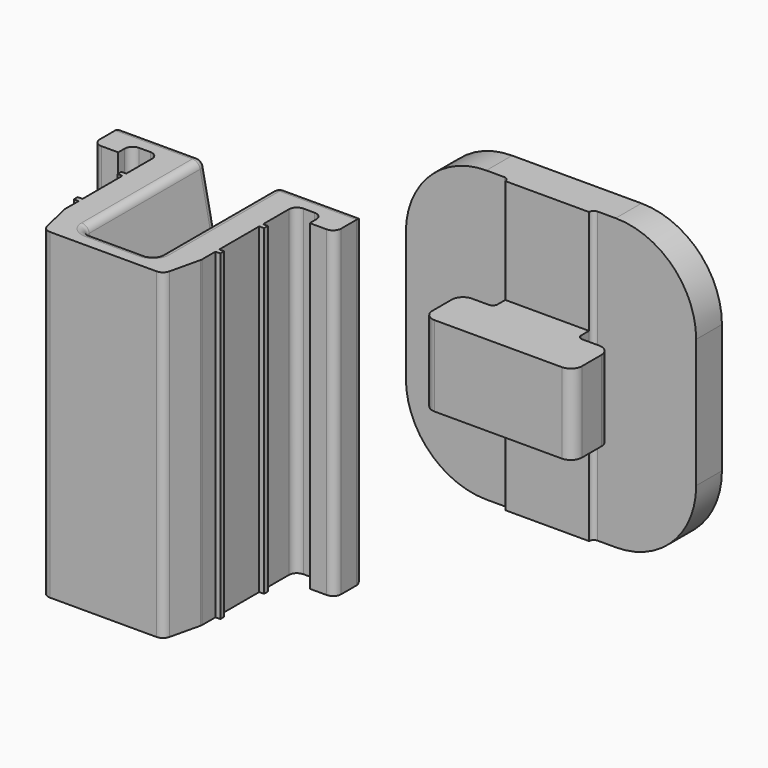
from build123d import *

# Parameters (mm, degrees)
F1_DEPTH = 20
F3_DEPTH = 9.6
F4_R     = 0.5
F6_DEPTH = 2.5
F7_DEPTH = 9
F8_DEPTH = 2
F9_R     = 5


# Not quite as in the source:
# - a feature names something its author has since deleted; it is built from what else it names


with BuildPart() as f1:
    # F0 (on Top) → F1 (new body)
    with BuildSketch(Plane.XY):
        Polygon((-4.25, 2.3122045677), (-3.7083309144, 0), (3.7083309144, 0), (4.25, 2.3122045677), (4.25, 3.4), (4.55, 3.4), (4.55, 3.7), (4.25, 3.7), (4.25, 6.8), (4.55, 6.8), (4.55, 7.1), (4.25, 7.1), (4.25, 9.6), (5.95, 9.6), (5.95, 8.6), (7.5, 8.6), (7.5, 10.8), (1.3, 10.8), (1.3, 1.2), (-1.3, 1.2), (-1.3, 10.8), (-7.5, 10.8), (-7.5, 8.6), (-5.95, 8.6), (-5.95, 9.6), (-4.25, 9.6), (-4.25, 7.1), (-4.55, 7.1), (-4.55, 6.8), (-4.25, 6.8), (-4.25, 3.7), (-4.55, 3.7), (-4.55, 3.4), (-4.25, 3.4), align=None)
    extrude(amount=F1_DEPTH)

    # F2 (on face) → F3 (cut)
    with BuildSketch(Plane(origin=(0, 10.8, 0), x_dir=(-1, 0, 0), z_dir=(0, 1, 0))):
        Polygon((2.3, 0), (1.3, 5), (1.3, 0), align=None)
        Polygon((-2.3, 0), (-1.3, 0), (-1.3, 5), align=None)
        Polygon((-2.3, 20), (-1.3, 15), (-1.3, 20), align=None)
        Polygon((2.3, 20), (1.3, 20), (1.3, 15), align=None)
    extrude(amount=-F3_DEPTH, mode=Mode.SUBTRACT)

    # F4
    f4_edges = [f1.edges().sort_by_distance(p)[0] for p in [
        (4.9, 10.8, 0),
        (1.8, 10.8, 2.5),
        (1.3, 10.8, 10),
        (1.8, 10.8, 17.5),
        (4.9, 10.8, 20),
        (7.5, 10.8, 10),
        (-1.8, 10.8, 2.5),
        (-4.9, 10.8, 0),
        (-7.5, 10.8, 10),
        (-4.9, 10.8, 20),
        (-1.8, 10.8, 17.5),
        (-1.3, 10.8, 10),
        (-2.3, 6, 0),
        (-1.3, 6, 5),
        (-1.8, 1.2, 2.5),
        (1.3, 6, 5),
        (2.3, 6, 0),
        (1.8, 1.2, 2.5),
        (2.3, 6, 20),
        (1.3, 6, 15),
        (1.8, 1.2, 17.5),
        (-1.3, 6, 15),
        (-2.3, 6, 20),
        (-1.8, 1.2, 17.5),
        (-4.25, 9.6, 10),
        (-5.95, 9.6, 10),
        (4.25, 9.6, 10),
        (5.95, 9.6, 10),
        (-7.5, 8.6, 10),
        (7.5, 8.6, 10),
        (3.708331, 0, 10),
        (4.25, 2.312205, 10),
        (-4.25, 2.312205, 10),
        (-3.708331, 0, 10),
        (0, 1.2, 20),
        (-1.3, 1.2, 10),
        (1.3, 1.2, 10),
        (0, 1.2, 0),
    ]]
    fillet(f4_edges, radius=F4_R)


with BuildPart() as f6:
    # F5 (on Top) → F6 (new body, symmetric)
    with BuildSketch(Plane.XY):
        with BuildLine():
            Line((-2.9, 33.5718078229), (-3.95, 33.5718078229))
            ThreePointArc((-3.95, 33.5718078229), (-4.4449747468, 33.3667825697), (-4.65, 32.8718078229))
            Line((-4.65, 32.8718078229), (-4.65, 31.3718078229))
            ThreePointArc((-4.65, 31.3718078229), (-4.4449747468, 30.876833076), (-3.95, 30.6718078229))
            Line((-3.95, 30.6718078229), (3.95, 30.6718078229))
            ThreePointArc((3.95, 30.6718078229), (4.4449747468, 30.876833076), (4.65, 31.3718078229))
            Line((4.65, 31.3718078229), (4.65, 32.8718078229))
            ThreePointArc((4.65, 32.8718078229), (4.4449747468, 33.3667825697), (3.95, 33.5718078229))
            Line((3.95, 33.5718078229), (2.9, 33.5718078229))
            ThreePointArc((2.9, 33.5718078229), (2.6878679656, 33.6596757885), (2.6, 33.8718078229))
            Line((2.6, 33.8718078229), (2.6, 34.4718078229))
            Line((2.6, 34.4718078229), (-2.6, 34.4718078229))
            Line((-2.6, 34.4718078229), (-2.6, 33.8718078229))
            ThreePointArc((-2.6, 33.8718078229), (-2.6878679656, 33.6596757885), (-2.9, 33.5718078229))
        make_face()
        with BuildLine():
            ThreePointArc((-2.9, 34.7718078229), (-2.6878679656, 34.6839398572), (-2.6, 34.4718078229))
            Line((-2.6, 34.4718078229), (2.6, 34.4718078229))
            ThreePointArc((2.6, 34.4718078229), (2.6878679656, 34.6839398572), (2.9, 34.7718078229))
            Line((2.9, 34.7718078229), (2.75, 34.7718078229))
            Line((2.75, 34.7718078229), (-2.75, 34.7718078229))
            Line((-2.75, 34.7718078229), (-2.9, 34.7718078229))
        make_face()
    extrude(amount=F6_DEPTH, both=True)

    # F5 (on Top) → F7 (join, symmetric)
    with BuildSketch(Plane.XY):
        Polygon((-9.0172681957, 34.7718078229), (-2.9, 34.7718078229), (-2.75, 34.7718078229), (2.75, 34.7718078229), (2.9, 34.7718078229), (9.0172681957, 34.7718078229), (9.0172681957, 36.7718078229), (5.5, 36.7718078229), (2.5, 36.7718078229), (-2.5, 36.7718078229), (-5.5, 36.7718078229), (-9.0172681957, 36.7718078229), align=None)
        with BuildLine():
            ThreePointArc((-2.9, 34.7718078229), (-2.6878679656, 34.6839398572), (-2.6, 34.4718078229))
            Line((-2.6, 34.4718078229), (2.6, 34.4718078229))
            ThreePointArc((2.6, 34.4718078229), (2.6878679656, 34.6839398572), (2.9, 34.7718078229))
            Line((2.9, 34.7718078229), (2.75, 34.7718078229))
            Line((2.75, 34.7718078229), (-2.75, 34.7718078229))
            Line((-2.75, 34.7718078229), (-2.9, 34.7718078229))
        make_face()
    extrude(amount=F7_DEPTH, both=True)

    # F5 (on Top) → F8 (join, symmetric)
    with BuildSketch(Plane.XY):
        with BuildLine():
            Line((-5.5, 38.7718078229), (-5.5, 36.7718078229))
            Line((-5.5, 36.7718078229), (-2.5, 36.7718078229))
            Line((-2.5, 36.7718078229), (-2.5, 38.7718078229))
            ThreePointArc((-2.5, 38.7718078229), (0, 41.2718078229), (2.5, 38.7718078229))
            Line((2.5, 38.7718078229), (2.5, 36.7718078229))
            Line((2.5, 36.7718078229), (5.5, 36.7718078229))
            Line((5.5, 36.7718078229), (5.5, 38.7718078229))
            ThreePointArc((5.5, 38.7718078229), (0, 44.2718078229), (-5.5, 38.7718078229))
        make_face()
    extrude(amount=F8_DEPTH, both=True)

    # F9
    f9_edges = [f6.edges().sort_by_distance(p)[0] for p in [
        (-9.017268, 35.771808, 9),
        (-9.017268, 35.771808, -9),
        (9.017268, 35.771808, 9),
        (9.017268, 35.771808, -9),
    ]]
    fillet(f9_edges, radius=F9_R)


solid = Compound([f1.part, f6.part])
